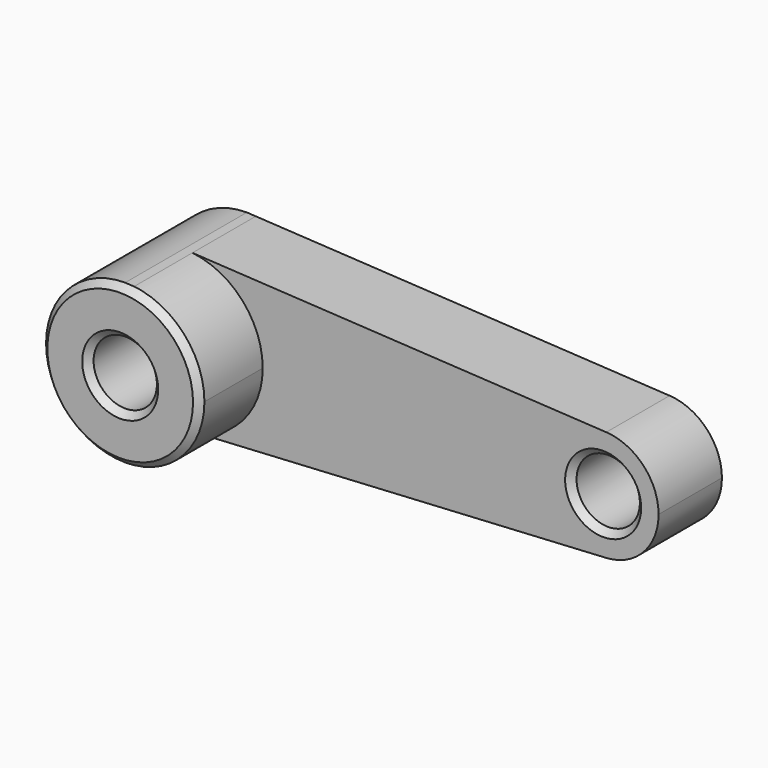
from build123d import *

# Parameters (mm, degrees)
F0_R        = 10
F1_DEPTH    = 25
F2_DEPTH    = 50
F3_T4_ANGLE = 203.6133668192
F3_T8_ANGLE = 190.697258089


# Not quite as in the source:
# - a fillet or chamfer that OpenCascade refuses, or shapes differently, is made with other operations: its cross-section is extruded or revolved along the edge and cut away or added


with BuildPart() as f1:
    # F0 (on Front) → F1 (new body)
    with BuildSketch(Plane.XZ):
        with BuildLine():
            Line((2.8107571296, 24.8414903812), (0, 25))
            ThreePointArc((0, 25), (-25, 0), (0, -25))
            Line((0, -25), (2.8107571296, -24.8414903812))
            ThreePointArc((2.8107571296, -24.8414903812), (18.6449581421, -16.6542948179), (25, 0))
            ThreePointArc((25, 0), (18.6449581421, 16.6542948179), (2.8107571296, 24.8414903812))
        make_face()
        Circle(F0_R, mode=Mode.SUBTRACT)
        with BuildLine():
            Line((133.4853280749, 17.4722387972), (2.8107571296, 24.8414903812))
            ThreePointArc((2.8107571296, 24.8414903812), (18.6449581421, 16.6542948179), (25, 0))
            ThreePointArc((25, 0), (18.6449581421, -16.6542948179), (2.8107571296, -24.8414903812))
            Line((2.8107571296, -24.8414903812), (133.4853280749, -17.4722387972))
            ThreePointArc((133.4853280749, -17.4722387972), (115, 0), (133.4853280749, 17.4722387972))
        make_face()
        with BuildLine():
            ThreePointArc((150, 0), (145.2179644855, 12.0209558415), (133.4853280749, 17.4722387972))
            ThreePointArc((133.4853280749, 17.4722387972), (115, 0), (133.4853280749, -17.4722387972))
            ThreePointArc((133.4853280749, -17.4722387972), (145.2179644855, -12.0209558415), (150, 0))
        make_face()
        with Locations((132.5, 0)):
            Circle(F0_R, mode=Mode.SUBTRACT)
    extrude(amount=F1_DEPTH)

    # F0 (on Front) → F2 (join)
    with BuildSketch(Plane.XZ):
        with BuildLine():
            Line((2.8107571296, 24.8414903812), (0, 25))
            ThreePointArc((0, 25), (-25, 0), (0, -25))
            Line((0, -25), (2.8107571296, -24.8414903812))
            ThreePointArc((2.8107571296, -24.8414903812), (18.6449581421, -16.6542948179), (25, 0))
            ThreePointArc((25, 0), (18.6449581421, 16.6542948179), (2.8107571296, 24.8414903812))
        make_face()
        Circle(F0_R, mode=Mode.SUBTRACT)
    extrude(amount=F2_DEPTH)

    # F3: chamfer of 2 on 4 edges, made by hand

    # F3_s1 → F3_t2 (revolve, cut)
    with BuildSketch(Plane.XY):
        Polygon((10, -48), (12, -50), (10, -50), align=None)
    revolve(axis=Axis((0, -50, 0), (0, -1, 0)), mode=Mode.SUBTRACT)

    # F3_s3 → F3_t4 (revolve, cut)
    with BuildSketch(Plane(origin=(0, 0, 0), x_dir=(0, 1, 0), z_dir=(0.9788435281, 0, -0.2046102329))):
        Polygon((-48, 25), (-50, 23), (-50, 25), align=None)
    revolve(axis=Axis((0, -50, 0), (0, -1, 0)), revolution_arc=F3_T4_ANGLE, mode=Mode.SUBTRACT)

    # F3_s5 → F3_t6 (revolve, cut)
    with BuildSketch(Plane.XY):
        Polygon((142.5, -23), (144.5, -25), (142.5, -25), align=None)
    revolve(axis=Axis((132.5, -25, 0), (0, -1, 0)), mode=Mode.SUBTRACT)

    # F3_s7 → F3_t8 (revolve, cut)
    with BuildSketch(Plane(origin=(0, 0, 0), x_dir=(0, 1, 0), z_dir=(-0.9956459412, 0, -0.0932156624))):
        Polygon((-48, -25), (-50, -23), (-50, -25), align=None)
    revolve(axis=Axis((0, -50, 0), (0, 1, 0)), revolution_arc=F3_T8_ANGLE, mode=Mode.SUBTRACT)


solid = f1.part
